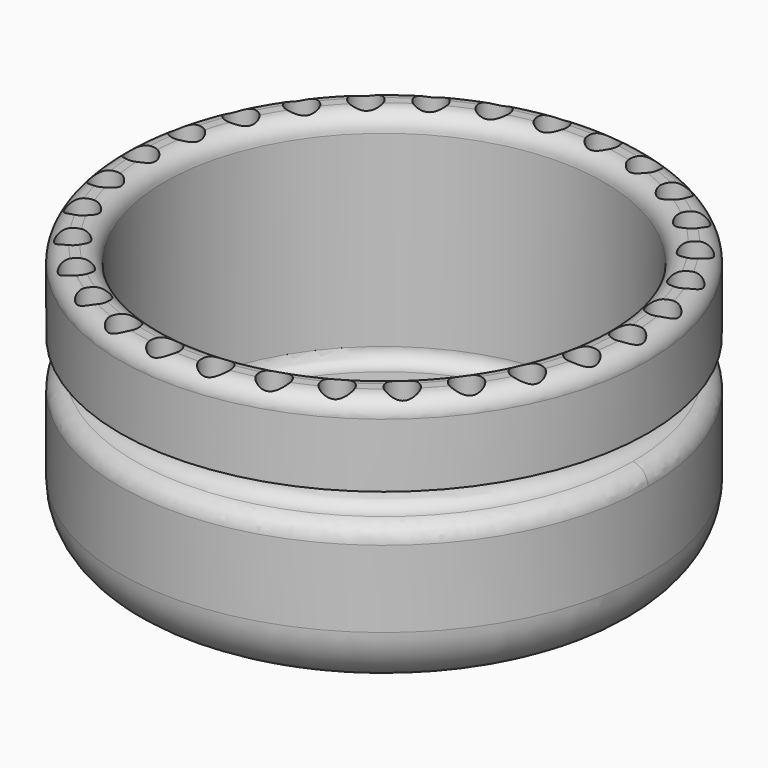
from build123d import *

# Parameters (mm, degrees)
F0_R     = 45
F1_DEPTH = 45
F2_R     = 10
F3_T     = -7.5
F5_R     = 2.5
F6_DEPTH = 15
F7_R     = 3
F9_R     = 3


# Not quite as in the source:
# - a fillet or chamfer that OpenCascade refuses, or shapes differently, is made with other operations: its cross-section is extruded or revolved along the edge and cut away or added


with BuildPart() as f1:
    # F0 (on Top) → F1 (new body)
    with BuildSketch(Plane.XY):
        Circle(F0_R)
    extrude(amount=F1_DEPTH)

    # F2
    f2_edges = [f1.edges().sort_by_distance(p)[0] for p in [
        (-45, 0, 0),
    ]]
    fillet(f2_edges, radius=F2_R)

    # F3
    f3_openings = [f1.faces().sort_by_distance(p)[0] for p in [
        (0, 0, 45),
    ]]
    offset(amount=F3_T, openings=f3_openings)

    # F5 (on offset) → F6 (cut)
    with BuildSketch(Plane.XY.offset(45)):
        with Locations((-41.5040434727, 0)):
            Circle(F5_R)
        with Locations((-40.5970805436, -8.6291758542)):
            Circle(F5_R)
        with Locations((-37.9158303883, -16.8812153162)):
            Circle(F5_R)
        with Locations((-33.5774765047, -24.3954646638)):
            Circle(F5_R)
        with Locations((-27.7716257752, -30.8435151431)):
            Circle(F5_R)
        with Locations((-20.7520217364, -35.9435560071)):
            Circle(F5_R)
        with Locations((-12.8254547683, -39.4726909973)):
            Circle(F5_R)
        with Locations((-4.3383538836, -41.2766799799)):
            Circle(F5_R)
        with Locations((4.3383538836, -41.2766799799)):
            Circle(F5_R)
        with Locations((12.8254547683, -39.4726909973)):
            Circle(F5_R)
        with Locations((20.7520217364, -35.9435560071)):
            Circle(F5_R)
        with Locations((27.7716257752, -30.8435151431)):
            Circle(F5_R)
        with Locations((33.5774765047, -24.3954646638)):
            Circle(F5_R)
        with Locations((37.9158303883, -16.8812153162)):
            Circle(F5_R)
        with Locations((40.5970805436, -8.6291758542)):
            Circle(F5_R)
        with Locations((41.5040434727, 0)):
            Circle(F5_R)
        with Locations((40.5970805436, 8.6291758542)):
            Circle(F5_R)
        with Locations((37.9158303883, 16.8812153162)):
            Circle(F5_R)
        with Locations((33.5774765047, 24.3954646638)):
            Circle(F5_R)
        with Locations((27.7716257752, 30.8435151431)):
            Circle(F5_R)
        with Locations((20.7520217364, 35.9435560071)):
            Circle(F5_R)
        with Locations((12.8254547683, 39.4726909973)):
            Circle(F5_R)
        with Locations((4.3383538836, 41.2766799799)):
            Circle(F5_R)
        with Locations((-4.3383538836, 41.2766799799)):
            Circle(F5_R)
        with Locations((-12.8254547683, 39.4726909973)):
            Circle(F5_R)
        with Locations((-20.7520217364, 35.9435560071)):
            Circle(F5_R)
        with Locations((-27.7716257752, 30.8435151431)):
            Circle(F5_R)
        with Locations((-33.5774765047, 24.3954646638)):
            Circle(F5_R)
        with Locations((-37.9158303883, 16.8812153162)):
            Circle(F5_R)
        with Locations((-40.5970805436, 8.6291758542)):
            Circle(F5_R)
    extrude(amount=-F6_DEPTH, mode=Mode.SUBTRACT)

    # F7 (on Front) → F8 (revolve, cut)
    with BuildSketch(Plane.XZ):
        with Locations((-42.8564883769, 29.0280934423)):
            Circle(F7_R)
    revolve(axis=Axis((0, 0, 21.2123766541), (0, 0, 1)), mode=Mode.SUBTRACT)

    # F9
    f9_edges = [f1.edges().sort_by_distance(p)[0] for p in [
        (-45, 0, 10),
        (45, 0, 18.464599),
        (0, -45, 26.929199),
        (0, 45, 26.929199),
    ]]
    fillet(f9_edges, radius=F9_R)

    # F10: fillet of radius 3 on 2 edges, made by hand

    # F10_s1 → F10_t2 (revolve, cut)
    with BuildSketch(Plane.XZ):
        with BuildLine():
            ThreePointArc((45, 42), (44.1213203436, 44.1213203436), (42, 45))
            Line((42, 45), (45, 45))
            Line((45, 45), (45, 42))
        make_face()
    revolve(axis=Axis((0, 0, 45), (0, 0, 1)), mode=Mode.SUBTRACT)

    # F10_s3 → F10_t4 (revolve, cut)
    with BuildSketch(Plane.XZ):
        with BuildLine():
            ThreePointArc((40.5, 45), (38.3786796564, 44.1213203436), (37.5, 42))
            Line((37.5, 42), (37.5, 45))
            Line((37.5, 45), (40.5, 45))
        make_face()
    revolve(axis=Axis((0, 0, 45), (0, 0, 1)), mode=Mode.SUBTRACT)


solid = f1.part
